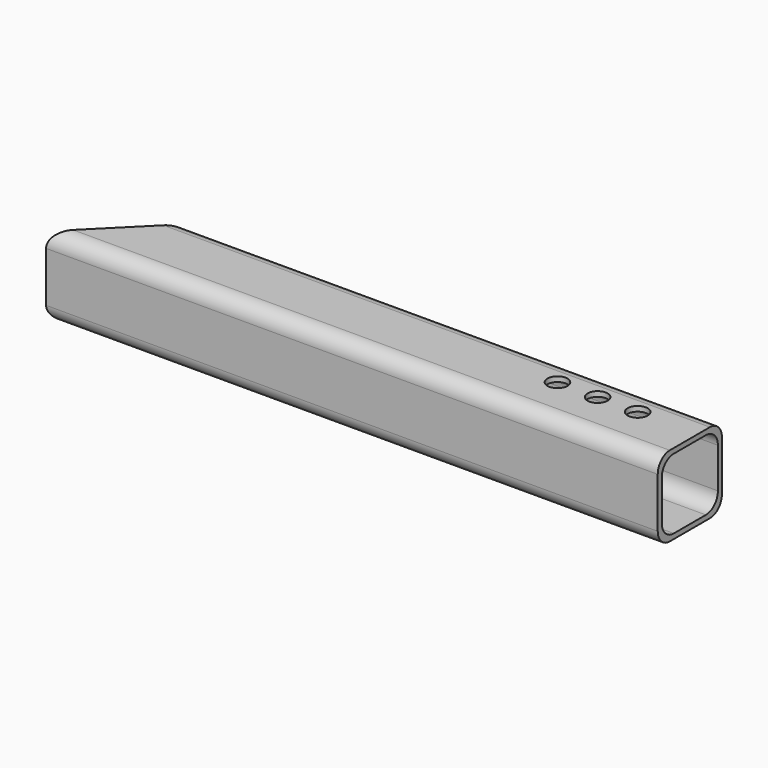
from build123d import *

# Parameters (mm, degrees)
F0_W     = 50.8
F0_H     = 50.8
F1_DEPTH = 387.35
F2_SIZE  = 50.79999
F3_W     = 44.45
F3_H     = 44.45
F4_DEPTH = 876.3
F5_R     = 9.525
F7_D     = 12.7
F7_DEPTH = 127
F7_TIP   = 3.8154649308


# Not quite as in the source:
# - a fillet or chamfer is up to 0.001 mm smaller than in the source, because OpenCascade refuses the exact size


with BuildPart() as f1:
    # F0 (on Right) → F1 (new body)
    with BuildSketch(Plane.YZ):
        with Locations((25.4, 25.4)):
            Rectangle(F0_W, F0_H)
    extrude(amount=-F1_DEPTH)

    # F2 (size 50.8 in the source; OpenCascade refuses exactly that, so slightly less here)
    f2_edges = [f1.edges().sort_by_distance(p)[0] for p in [
        (-387.35, 50.8, 25.4),
    ]]
    chamfer(f2_edges, length=F2_SIZE)

    # F3 (on face) → F4 (cut)
    with BuildSketch(Plane.YZ):
        with Locations((25.4, 25.4)):
            Rectangle(F3_W, F3_H)
    extrude(amount=-F4_DEPTH, mode=Mode.SUBTRACT)

    # F5
    f5_edges = [f1.edges().sort_by_distance(p)[0] for p in [
        (-192.087505, 3.175, 3.175),
        (-169.862505, 47.625, 3.175),
        (-169.862505, 47.625, 47.625),
        (-192.087505, 3.175, 47.625),
        (-168.275005, 50.8, 0),
        (-168.275005, 50.8, 50.8),
        (-193.675, 0, 50.8),
        (-193.675, 0, 0),
    ]]
    fillet(f5_edges, radius=F5_R)

    # F7
    with Locations(Plane(origin=(0, 0, 0), x_dir=(1, 0, 0), z_dir=(0, 0, -1))):
        with Locations((-38.1, -31.75), (-63.5, -31.75), (-88.9, -31.75)):
            Hole(F7_D / 2, depth=F7_DEPTH)
            with Locations((0, 0, -(F7_DEPTH + F7_TIP / 2))):  # 118° drill point
                Cone(0, F7_D / 2, F7_TIP, mode=Mode.SUBTRACT)


solid = f1.part
